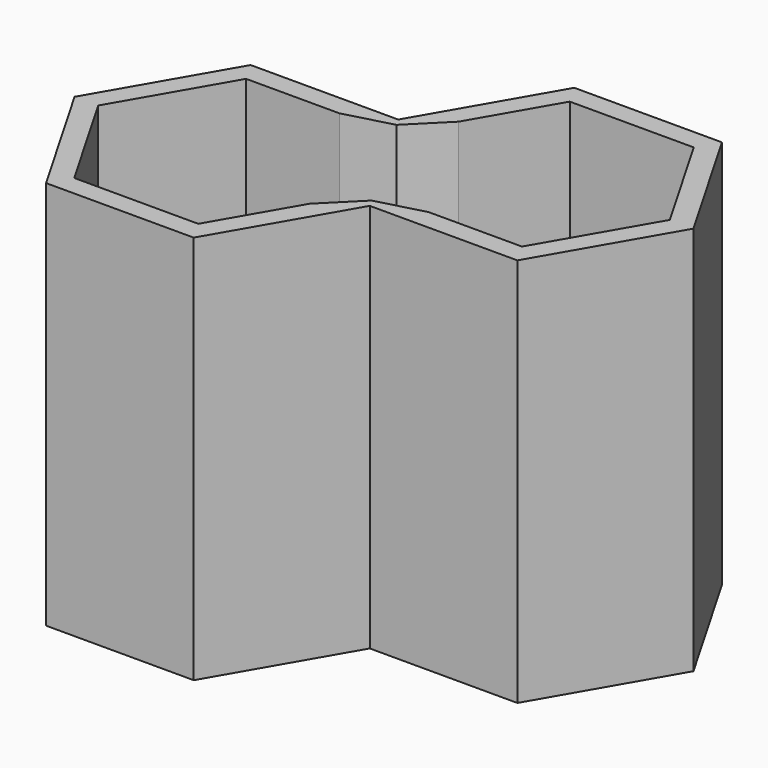
from build123d import *

# Parameters (mm, degrees)
F1_DEPTH    = 38.1
F2_T1_DEPTH = 53.6803294212


# Not quite as in the source:
# - a fillet or chamfer that OpenCascade refuses, or shapes differently, is made with other operations: its cross-section is extruded or revolved along the edge and cut away or added


with BuildPart() as f1:
    # F0 (on Top) → F1 (new body)
    with BuildSketch(Plane.XY):
        Polygon((-7.2168783649, -12.5), (7.2168783649, -12.5), (14.4337567297, 0), (28.8675134595, 0), (36.0843918244, 12.5), (28.8675134595, 25), (14.4337567297, 25), (7.2168783649, 12.5), (-7.2168783649, 12.5), (-14.4337567297, 0), align=None)
        Polygon((12.124355653, 0), (6.0621778265, -10.5), (-6.0621778265, -10.5), (-12.124355653, 0), (-6.0621778265, 10.5), (6.0621778265, 10.5), (9.5262794416, 12.5), (15.5884572681, 23), (27.7128129211, 23), (33.7749907476, 12.5), (27.7128129211, 2), (15.5884572681, 2), align=None, mode=Mode.SUBTRACT)
    extrude(amount=F1_DEPTH)

    # F2: chamfer of 3 on 4 edges, made by hand

    # F2_s2 → F2_t1 (cut)
    with BuildSketch(Plane.XY.offset(-7.7901647106)):
        Polygon((3.0621778265, 10.5), (8.6602540378, 12), (6.0621778265, 10.5), align=None)
        Polygon((6.9282032303, 11), (11.0262794416, 15.0980762114), (9.5262794416, 12.5), align=None)
        Polygon((14.7224318643, 1.5), (10.624355653, -2.5980762114), (12.124355653, 0), align=None)
        Polygon((18.5884572681, 2), (12.9903810568, 0.5), (15.5884572681, 2), align=None)
    extrude(amount=F2_T1_DEPTH, mode=Mode.SUBTRACT)


solid = f1.part
